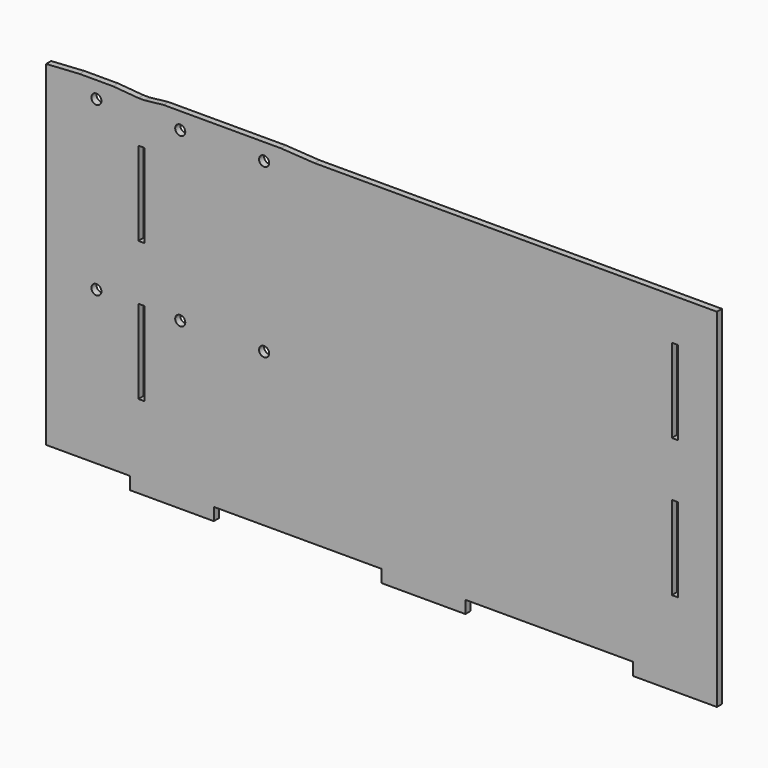
from build123d import *

# Parameters (mm, degrees)
F1_DEPTH  = 3.75
F2_W      = 3.75
F2_H      = 50
F3_DEPTH  = 3.75
F4_W      = 20
F4_H      = 3.75
F5_DEPTH  = 1.25
F7_D      = 6
F7_DEPTH  = 4
F7_TIP    = 1.8025818571
F8_W      = 30
F8_H      = 1.25
F9_DEPTH  = 3.75
F10_W     = 3.75
F10_H     = 50
F11_DEPTH = 3.75


# Not quite as in the source:
# - a feature names something its author has since deleted; it is built from what else it names


with BuildPart() as f1:
    # F0 (on Front) → F1 (new body)
    with BuildSketch(Plane.XZ):
        Polygon((50, -7.5), (50, 0), (150, 0), (150, -7.5), (200, -7.5), (200, 0), (300, 0), (300, -7.5), (350, -7.5), (350, 0), (350, 200), (0, 200), (-50, 200), (-50, 0), (0, 0), (0, -7.5), align=None)
    extrude(amount=F1_DEPTH)

    # F2 (on face) → F3 (cut)
    with BuildSketch(Plane.XZ.offset(3.75)):
        with Locations((325, 150)):
            Rectangle(F2_W, F2_H)
        with Locations((325, 67.5)):
            Rectangle(F2_W, F2_H)
    extrude(amount=-F3_DEPTH, mode=Mode.SUBTRACT)

    # F4 (on face) → F5 (join)
    with BuildSketch(Plane.XY.offset(200)):
        with Locations((80, -1.875)):
            Rectangle(F4_W, F4_H)
        with Locations((30, -1.875)):
            Rectangle(F4_W, F4_H)
        with Locations((-20, -1.875)):
            Rectangle(F4_W, F4_H)
    extrude(amount=F5_DEPTH)

    # F7
    with Locations(Plane(origin=(0, 0, 0), x_dir=(-1, 0, 0), z_dir=(0, 1, 0))):
        with Locations((-80, 91.25), (-80, 191.25), (-30, 91.25), (20, 91.25), (20, 191.25), (-30, 191.25)):
            Hole(F7_D / 2, depth=F7_DEPTH)
            with Locations((0, 0, -(F7_DEPTH + F7_TIP / 2))):  # 118° drill point
                Cone(0, F7_D / 2, F7_TIP, mode=Mode.SUBTRACT)

    # F8 (on face) → F9 (join)
    with BuildSketch(Plane(origin=(0, 0, 0), x_dir=(-1, 0, 0), z_dir=(0, 1, 0))):
        with Locations((-55, 200.625)):
            Rectangle(F8_W, F8_H)
        Polygon((30, 201.25), (30, 200), (50, 200), align=None)
        Polygon((-90, 200), (-90, 201.25), (-110, 200), align=None)
        Polygon((10, 201.25), (-5, 200), (10, 200), align=None)
        Polygon((-8.75, 200), (-20, 201.25), (-20, 200), align=None)
    extrude(amount=-F9_DEPTH)

    # F10 (on face) → F11 (cut)
    with BuildSketch(Plane(origin=(0, 0, 0), x_dir=(-1, 0, 0), z_dir=(0, 1, 0))):
        with Locations((-6.875, 150)):
            Rectangle(F10_W, F10_H)
        with Locations((-6.875, 67)):
            Rectangle(F10_W, F10_H)
    extrude(amount=-F11_DEPTH, mode=Mode.SUBTRACT)


solid = f1.part
